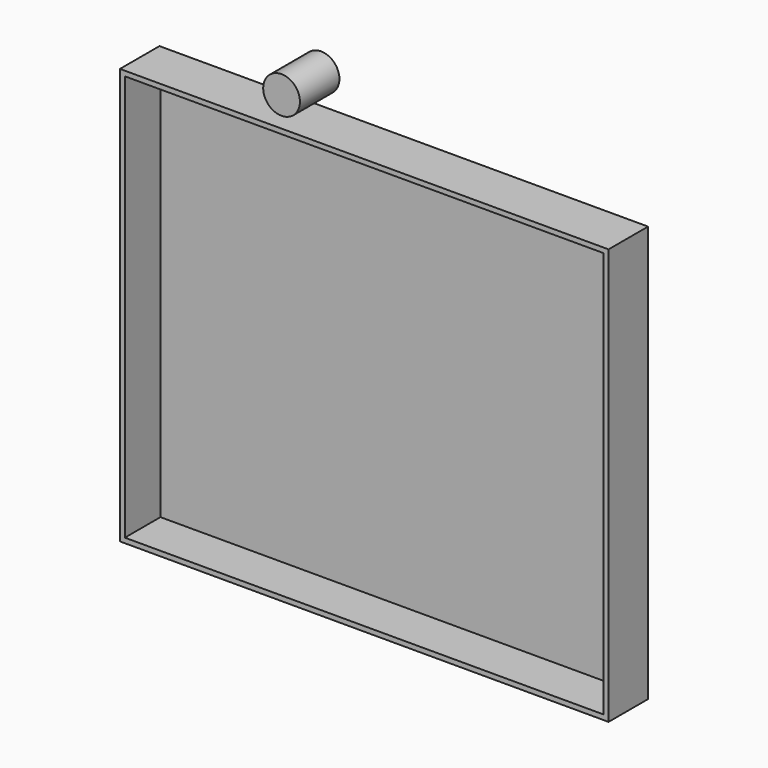
from build123d import *

# Parameters (mm, degrees)
F0_W     = 251.3852417469
F0_H     = 214.0397690237
F2_DEPTH = 25.4
F3_T     = -2.54
F4_R     = 9.4419076599
F5_DEPTH = 25.4


# Not quite as in the source:
# - the program builds the solid bodies; features that only make, move or delete a surface that nothing else refers to are left out


with BuildPart() as f2:
    # F0 (on Front) → F2 (new body)
    with BuildSketch(Plane.XZ):
        with Locations((-480.2153557539, -85.1046163589)):
            Rectangle(F0_W, F0_H)
    extrude(amount=F2_DEPTH)

    # F3
    f3_openings = [f2.faces().sort_by_distance(p)[0] for p in [
        (-480.215356, -25.4, -85.104616),
    ]]
    offset(amount=F3_T, openings=f3_openings)


with BuildPart() as f5:
    # F4 (on face) → F5 (new body)
    with BuildSketch(Plane.XZ.offset(2.54)):
        with Locations((-520.7318067551, 38.8364158571)):
            Circle(F4_R)
    extrude(amount=F5_DEPTH)


solid = Compound([f2.part, f5.part])
